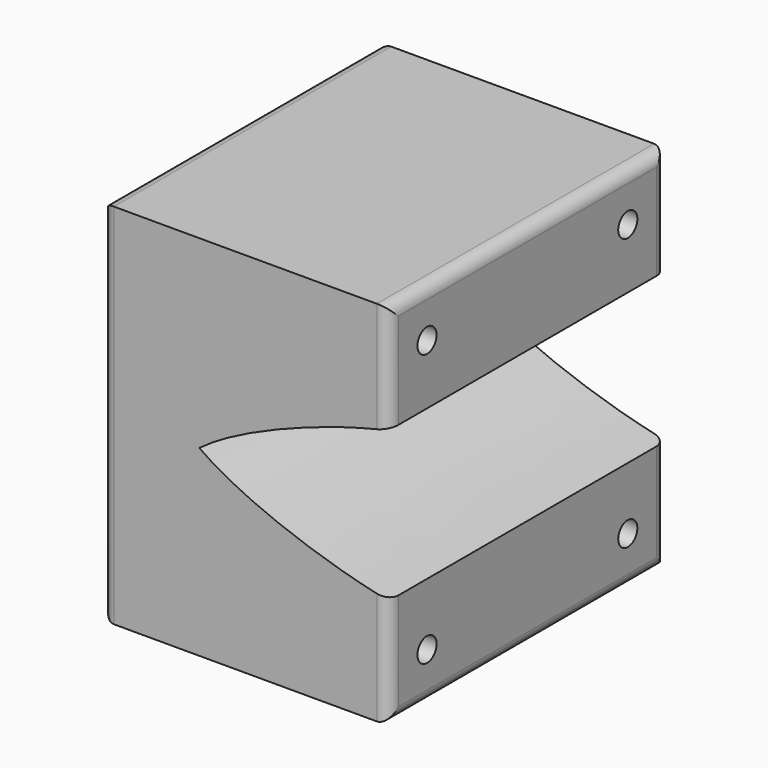
from build123d import *

# Parameters (mm, degrees)
F1_DEPTH       = 72.5
F3_D           = 5
F3_CBORE_D     = 10
F3_CBORE_DEPTH = 5
F4_R           = 2.5
F5_R           = 2.5


# Not quite as in the source:
# - ends of sketch curves that miss each other by under 0.0002 mm in the source are joined
# - the dataset's text gives a spline's control points without its knots; the knots are read off the source's solid


with BuildPart() as f1:
    # F0 (on Front) → F1 (new body)
    with BuildSketch(Plane.XZ):
        with BuildLine():
            add(Edge.make_bspline(
                [(-56.5881601574, 0.0419234738), (-55.5197950815, -0.7442946781), (-53.1301338185, -2.2933127374), (-48.9084685045, -4.5561843947), (-44.1859500973, -6.7339324001), (-39.1068883918, -8.7916644331), (-33.8193544964, -10.6897211609), (-29.3644227389, -12.1035605133), (-25.8455914341, -13.1126993817), (-22.383504382, -14.0327971877), (-19.4313477815, -14.7259719893), (-17.3706943762, -15.160741157), (-16.9593766332, -15.2455717325)],
                knots=[0, 0, 0, 0, 0.03125, 0.0625, 0.09375, 0.125, 0.15625, 0.1875, 0.203125, 0.21875, 0.25, 0.2578399244, 0.2578399244, 0.2578399244, 0.2578399244], degree=3))
            add(Edge.make_bspline(
                [(-56.5881601574, 0.0419234738), (-55.5355017666, 0.8486239051), (-53.1764131036, 2.443347048), (-48.9992069483, 4.7861572474), (-44.3187202519, 7.053077305), (-39.2793074327, 9.2063486815), (-34.0283660726, 11.2037109249), (-29.6007919855, 12.7012369201), (-26.1016179695, 13.7765699234), (-22.65755408, 14.761891198), (-19.6168305087, 15.5368665147), (-17.4672919643, 16.0305431026), (-16.9593493648, 16.1441983995)],
                knots=[1.43705e-05, 1.43705e-05, 1.43705e-05, 1.43705e-05, 0.03125, 0.0625, 0.09375, 0.125, 0.15625, 0.1875, 0.203125, 0.21875, 0.25, 0.2597438328, 0.2597438328, 0.2597438328, 0.2597438328], degree=3))
            Line((-16.9593493648, 16.1441983995), (-16.9593493648, 38.671177907))
            Line((-16.9593493648, 38.671177907), (-76.9551545382, 38.671177907))
            Line((-76.9551545382, 38.671177907), (-76.9551545382, -38.248822093))
            Line((-76.9551545382, -38.248822093), (-16.9593493648, -38.248822093))
            Line((-16.9593493648, -38.248822093), (-16.9593766332, -15.2455717325))
        make_face()
    extrude(amount=F1_DEPTH)

    # F3 (through all)
    with Locations(Plane(origin=(-76.9551545382, 0, 0), x_dir=(0, -1, 0), z_dir=(-1, 0, 0))):
        with Locations((10, 28.671177907), (62.5, 28.671177907), (62.5, -28.248822093), (10, -28.248822093)):
            CounterBoreHole(F3_D / 2, F3_CBORE_D / 2, F3_CBORE_DEPTH)

    # F4
    f4_edges = [f1.edges().sort_by_distance(p)[0] for p in [
        (-76.955155, -72.5, 0.211178),
        (-76.955155, -36.25, 38.671178),
        (-76.955155, 0, 0.211178),
        (-76.955155, -36.25, -38.248822),
    ]]
    fillet(f4_edges, radius=F4_R)

    # F5
    f5_edges = [f1.edges().sort_by_distance(p)[0] for p in [
        (-16.959349, -36.25, 38.671178),
        (-16.959349, -72.5, 27.407688),
        (-16.959349, 0, 27.407688),
        (-16.959363, 0, -26.747197),
        (-16.959349, -36.25, -38.248822),
        (-16.959363, -72.5, -26.747197),
    ]]
    fillet(f5_edges, radius=F5_R)


solid = f1.part
